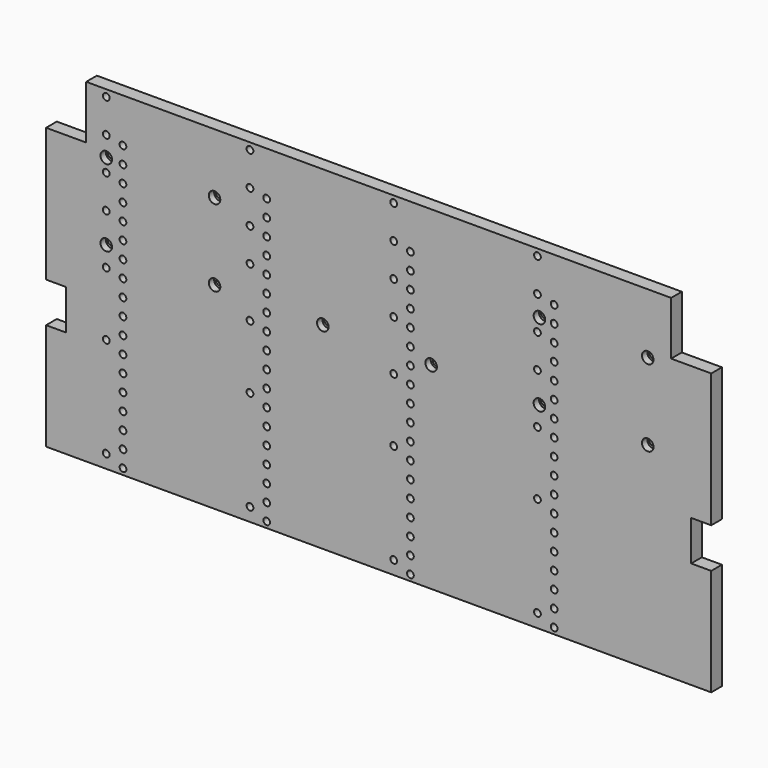
from build123d import *

# Parameters (mm, degrees)
F1_DEPTH       = 20
F3_D           = 11
F3_DEPTH       = 35
F3_CBORE_D     = 17.25
F3_CBORE_DEPTH = 10
F3_TIP         = 3.3047334047
F5_D           = 10.1
F7_D           = 10.1


# Not quite as in the source:
# - a feature names something its author has since deleted; it is built from what else it names


with BuildPart() as f1:
    # F0 (on Front) → F1 (new body)
    with BuildSketch(Plane.XZ):
        Polygon((-497.5, -250), (497.5, -250), (497.5, -90), (467.5, -90), (467.5, -30), (497.5, -30), (497.5, 170), (437.5, 170), (437.5, 250), (-437.5, 250), (-437.5, 170), (-497.5, 170), (-497.5, -30), (-467.5, -30), (-467.5, -90), (-497.5, -90), align=None)
    extrude(amount=-F1_DEPTH)

    # F3
    with Locations(Plane.XZ):
        with Locations((-83.5, 45), (-407.5, 160), (78.5, 45), (-407.5, 45), (240.5, 160), (-245.5, 160), (402.5, 45), (240.5, 45), (-245.5, 45), (402.5, 160)):
            CounterBoreHole(F3_D / 2, F3_CBORE_D / 2, F3_CBORE_DEPTH, depth=F3_DEPTH)
            with Locations((0, 0, -(F3_DEPTH + F3_TIP / 2))):  # 118° drill point
                Cone(0, F3_D / 2, F3_TIP, mode=Mode.SUBTRACT)

    # F5 (through all)
    with Locations(Plane.XZ):
        with Locations((-407.5, -80), (-407.5, 15), (-407.5, -230), (-407.5, 90), (-407.5, 240), (-407.5, 140), (-407.5, 190), (22.5, 190), (-192.5, 190), (237.5, 90), (-192.5, 15), (237.5, -80), (-192.5, -80), (-192.5, -230), (237.5, -230), (237.5, 190), (-192.5, 140), (22.5, -80), (22.5, 140), (-192.5, 240), (22.5, -230), (-192.5, 90), (237.5, 140), (237.5, 15), (237.5, 240), (22.5, 240), (22.5, 15), (22.5, 90)):
            Hole(F5_D / 2)

    # F7 (through all)
    with Locations(Plane.XZ):
        with Locations((47.5, -116), (262.5, -91), (-382.5, -166), (-167.5, -141), (-167.5, -16), (47.5, 9), (262.5, 9), (-167.5, -41), (47.5, -16), (-167.5, 34), (47.5, 59), (262.5, 59), (-167.5, 9), (47.5, 34), (262.5, 34), (-167.5, 84), (47.5, 109), (262.5, 109), (-167.5, 59), (47.5, 84), (262.5, 84), (262.5, 159), (-382.5, 59), (-167.5, 109), (47.5, 134), (262.5, 134), (-382.5, 84), (-382.5, 9), (-382.5, 34), (-382.5, -41), (-382.5, -16), (-382.5, -66), (-382.5, 159), (-382.5, 184), (-382.5, 109), (-382.5, 134), (47.5, -66), (-382.5, -141), (262.5, 184), (262.5, -41), (262.5, -216), (-167.5, 134), (-167.5, -91), (47.5, 159), (47.5, -91), (-382.5, -116), (47.5, -191), (262.5, -66), (262.5, -166), (-167.5, 184), (-167.5, -116), (-167.5, -216), (47.5, -41), (-382.5, -91), (47.5, -216), (262.5, -191), (262.5, -16), (-167.5, 159), (-167.5, -66), (47.5, 184), (47.5, -141), (262.5, -116), (-382.5, -191), (-167.5, -166), (47.5, -166), (262.5, -141), (-382.5, -216), (-167.5, -191), (-382.5, -241), (-167.5, -241), (47.5, -241), (262.5, -241)):
            Hole(F7_D / 2)


solid = f1.part
